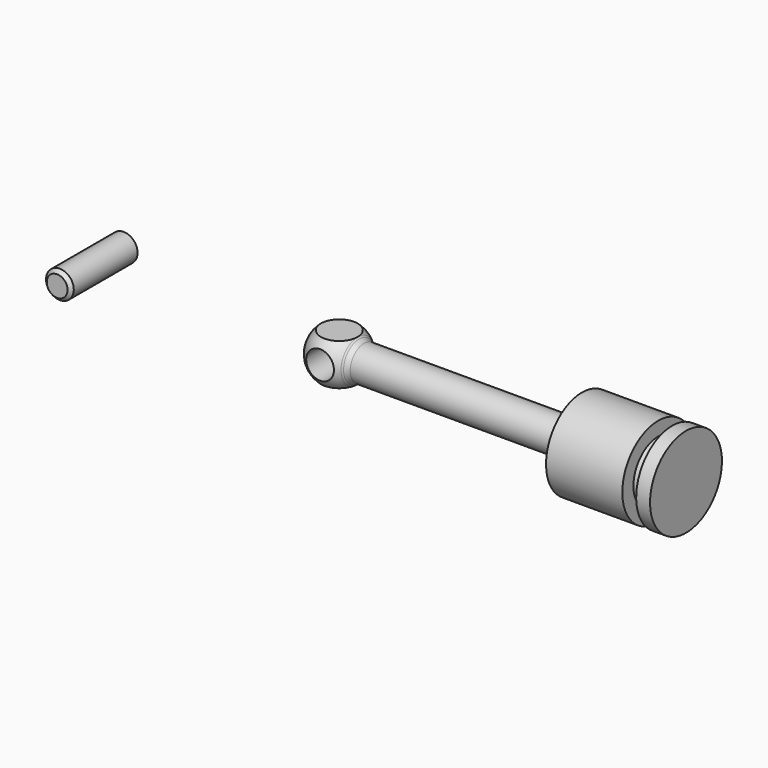
from build123d import *
from build123d import SkipClean  # not in build123d's __all__

# Parameters (mm, degrees)
F0_W     = 5
F0_H     = 2.5
F2_DEPTH = 12.5
F3_R     = 1
F4_W     = 2
F4_H     = 4.48
F0_R     = 2
F6_DEPTH = 12
F7_SIZE  = 0.5


with BuildPart() as f1:
    # F0 (on Front) → F1 (revolve)
    with BuildSketch(Plane.XZ):
        with BuildLine():
            ThreePointArc((2.6457513111, 3), (0, 4), (-2.6457513111, 3))
            Line((-2.6457513111, 3), (2.6457513111, 3))
        make_face()
        with BuildLine():
            ThreePointArc((-2, 0), (0, 2), (2, 0))
            Line((2, 0), (4, 0))
            ThreePointArc((4, 0), (3.7742546282, 1.3247648854), (3.1224989992, 2.5))
            ThreePointArc((3.1224989992, 2.5), (2.894940053, 2.7603119551), (2.6457513111, 3))
            Line((2.6457513111, 3), (-2.6457513111, 3))
            ThreePointArc((-2.6457513111, 3), (-3.6457513111, 1.6457513111), (-4, 0))
            Line((-4, 0), (-2, 0))
        make_face()
        with BuildLine():
            ThreePointArc((3.1224989992, 2.5), (3.7742546282, 1.3247648854), (4, 0))
            Line((4, 0), (35, 0))
            Line((35, 0), (35, 2.5))
            Line((35, 2.5), (3.1224989992, 2.5))
        make_face()
        with BuildLine():
            Line((-2, 0), (0, 0))
            Line((0, 0), (2, 0))
            ThreePointArc((2, 0), (0, 2), (-2, 0))
        make_face()
        with Locations((37.5, 1.25)):
            Rectangle(F0_W, F0_H)
    revolve(axis=Axis((25.0713285059, 0, 0), (1, 0, 0)))

    # F0 (on Front) → F2 (cut, symmetric)
    with BuildSketch(Plane.XZ):
        with BuildLine():
            ThreePointArc((2.6457513111, 3), (0, 4), (-2.6457513111, 3))
            Line((-2.6457513111, 3), (2.6457513111, 3))
        make_face()
        with BuildLine():
            Line((2.6457513111, -3), (-2.6457513111, -3))
            ThreePointArc((-2.6457513111, -3), (0, -4), (2.6457513111, -3))
        make_face()
        with BuildLine():
            Line((-2, 0), (0, 0))
            Line((0, 0), (2, 0))
            ThreePointArc((2, 0), (0, 2), (-2, 0))
        make_face()
        with BuildLine():
            Line((2, 0), (0, 0))
            Line((0, 0), (-2, 0))
            ThreePointArc((-2, 0), (0, -2), (2, 0))
        make_face()
    with SkipClean():  # cleaning this boolean's faces spoils the solid; the shape is the same uncleaned
        extrude(amount=F2_DEPTH, both=True, mode=Mode.SUBTRACT)

    # F3
    f3_edges = [f1.edges().sort_by_distance(p)[0] for p in [
        (3.122499, 0, -2.5),
    ]]
    fillet(f3_edges, radius=F3_R)


with BuildPart() as f5:
    # F4 (on Front) → F5 (revolve)
    with BuildSketch(Plane.XZ):
        Polygon((50, 6.48), (48, 6.48), (48, 4.48), (48, 0), (50, 0), align=None)
        with Locations((47, 2.24)):
            Rectangle(F4_W, F4_H)
        Polygon((35, 6.48), (35, 2.5), (40, 2.5), (40, 0), (46, 0), (46, 4.48), (46, 6.48), align=None)
    revolve(axis=Axis((42.5, 0, 0), (-1, 0, 0)))


with BuildPart() as f6:
    # F0 (on Front) → F6 (new body)
    with BuildSketch(Plane.XZ):
        with Locations((-31.0908816755, 3.3689432312)):
            Circle(F0_R)
    extrude(amount=F6_DEPTH)

    # F7
    f7_edges = [f6.edges().sort_by_distance(p)[0] for p in [
        (-33.090882, -12, 3.368943),
    ]]
    chamfer(f7_edges, length=F7_SIZE)


solid = Compound([f1.part, f5.part, f6.part])
